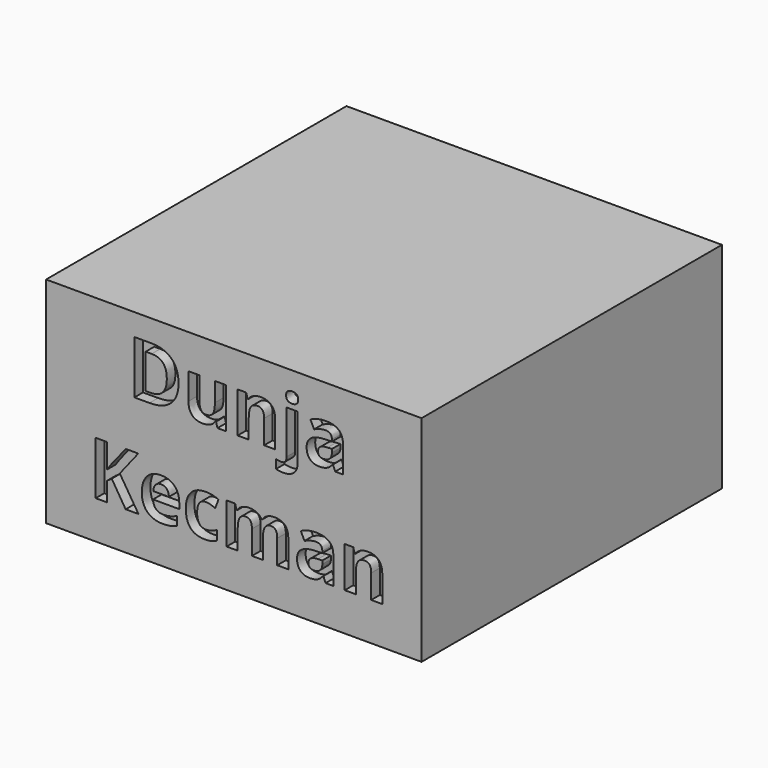
from build123d import *

# Parameters (mm, degrees)
F0_W         = 35
F0_H         = 35
F1_DEPTH     = 20
F2_TEXT_SIZE = 6.9444444444
F3_DEPTH     = 1


# Not quite as in the source:
# - Text() gives the source's letters only with a copy of the font that has no kerning and outlines rounded to 1/6400 em; it was checked with that copy


with BuildPart() as f1:
    # F0 (on Top) → F1 (new body)
    with BuildSketch(Plane.XY):
        with Locations((17.5, 17.5)):
            Rectangle(F0_W, F0_H)
    extrude(amount=F1_DEPTH)

    # F2 (on face) → F3 (cut)
    with BuildSketch(Plane.XZ):
        with Locations((7.6089409722, 13)):
            Text('Dunja', F2_TEXT_SIZE, font='Open Sans', font_style=FontStyle.BOLD, text_align=(TextAlign.LEFT, TextAlign.BOTTOM))
        with Locations((4, 3.5555555556)):
            Text('Kecman', F2_TEXT_SIZE, font='Open Sans', font_style=FontStyle.BOLD, text_align=(TextAlign.LEFT, TextAlign.BOTTOM))
    extrude(amount=-F3_DEPTH, mode=Mode.SUBTRACT)


solid = f1.part
